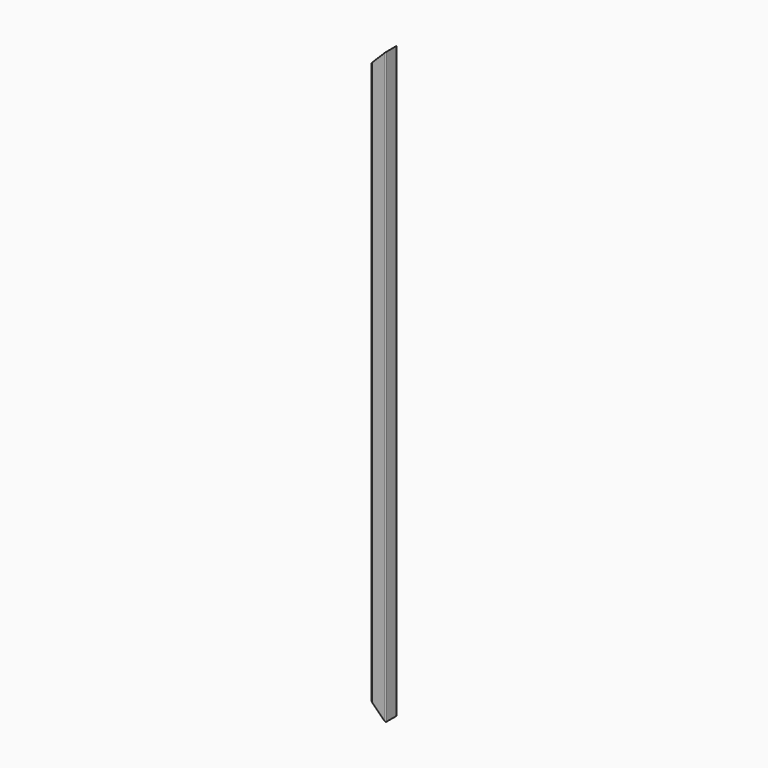
from build123d import *

# Parameters (mm, degrees)
F1_DEPTH      = 825
F3_DEPTH      = 20.001
F3_DEPTH_BACK = 20.001


# Not quite as in the source:
# - a pattern or mirror of a feature is missing from the dataset's text; its kind, count and spacing are read off the source's solid


with BuildPart() as f1:
    # F0 (on Top) → F1 (new body, symmetric)
    with BuildSketch(Plane.XY):
        with BuildLine():
            Line((17, 20), (-17, 20))
            ThreePointArc((-17, 20), (-19.1213203436, 19.1213203436), (-20, 17))
            Line((-20, 17), (-20, -17))
            ThreePointArc((-20, -17), (-19.1213203436, -19.1213203436), (-17, -20))
            Line((-17, -20), (17, -20))
            ThreePointArc((17, -20), (19.1213203436, -19.1213203436), (20, -17))
            Line((20, -17), (20, 17))
            ThreePointArc((20, 17), (19.1213203436, 19.1213203436), (17, 20))
        make_face()
        with BuildLine():
            ThreePointArc((-18, 17), (-17.7071067812, 17.7071067812), (-17, 18))
            Line((-17, 18), (17, 18))
            ThreePointArc((17, 18), (17.7071067812, 17.7071067812), (18, 17))
            Line((18, 17), (18, -17))
            ThreePointArc((18, -17), (17.7071067812, -17.7071067812), (17, -18))
            Line((17, -18), (-17, -18))
            ThreePointArc((-17, -18), (-17.7071067812, -17.7071067812), (-18, -17))
            Line((-18, -17), (-18, 17))
        make_face(mode=Mode.SUBTRACT)
    extrude(amount=F1_DEPTH, both=True)

    # F2 (on Front) → F3 (cut, two sides)
    with BuildSketch(Plane.XZ) as f3_sk:
        Polygon((20, 825), (-20, 825), (-20, 785), align=None)
    f3 = extrude(amount=-F3_DEPTH, mode=Mode.SUBTRACT) + extrude(f3_sk.sketch, amount=F3_DEPTH_BACK, mode=Mode.SUBTRACT)

    # F3_copies: F3 across plane
    add(f3.mirror(Plane(origin=(0, 0, 0), x_dir=(-1, 0, 0), z_dir=(0, 0, -1))), mode=Mode.SUBTRACT)


solid = f1.part
